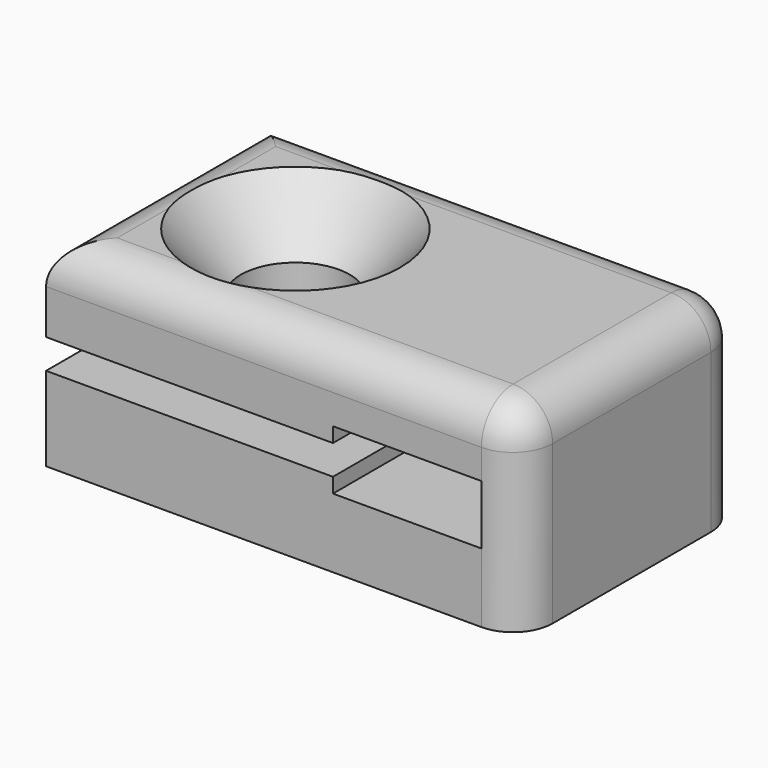
from build123d import *

# Parameters (mm, degrees)
F0_W           = 5
F0_H           = 7
F0_W_2         = 7
F1_DEPTH       = 5
F3_D           = 2.75
F3_CSINK_D     = 5.3
F3_CSINK_ANGLE = 82
F5_DEPTH       = 7
F6_T1_DEPTH    = 12
F6_T3_DEPTH    = 13.5
F6_T5_DEPTH    = 5
F6_T7_DEPTH    = 6.5
F6_S11_W       = 1
F6_S11_H       = 1
F6_T12_DEPTH   = 1
F6_S17_W       = 1
F6_S17_H       = 1
F6_T18_DEPTH   = 1


# Not quite as in the source:
# - a fillet or chamfer that OpenCascade refuses, or shapes differently, is made with other operations: its cross-section is extruded or revolved along the edge and cut away or added


with BuildPart() as f1:
    # F0 (on Top) → F1 (new body)
    with BuildSketch(Plane.XY):
        with Locations((3.5, 0)):
            Rectangle(F0_W, F0_H)
        with Locations((-2.5, 0)):
            Rectangle(F0_W_2, F0_H)
    extrude(amount=-F1_DEPTH)

    # F3 (through all)
    with Locations(Plane.XY):
        with Locations((-2.5, 0)):
            CounterSinkHole(F3_D / 2, F3_CSINK_D / 2, counter_sink_angle=F3_CSINK_ANGLE)

    # F4 (on face) → F5 (cut, through all)
    with BuildSketch(Plane.XZ.offset(3.5)):
        Polygon((1.25, -3.25), (4.9999998882, -3.25), (4.9999998882, -1.75), (1.25, -1.75), (1.25, -2.125), (-6, -2.125), (-6, -2.875), (1.25, -2.875), align=None)
    extrude(amount=-F5_DEPTH, mode=Mode.SUBTRACT)

    # F6: fillet of radius 1 on 6 edges, made by hand

    # F6_s2 → F6_t1 (cut)
    with BuildSketch(Plane.XZ.offset(-6)):
        with BuildLine():
            ThreePointArc((-5, 0), (-5.7071067812, -0.2928932188), (-6, -1))
            Line((-6, -1), (-6, 0))
            Line((-6, 0), (-5, 0))
        make_face()
    extrude(amount=F6_T1_DEPTH, mode=Mode.SUBTRACT)

    # F6_s4 → F6_t3 (cut)
    with BuildSketch(Plane.YZ.offset(-8.5)):
        with BuildLine():
            ThreePointArc((3.5, -1), (3.2071067812, -0.2928932188), (2.5, 0))
            Line((2.5, 0), (3.5, 0))
            Line((3.5, 0), (3.5, -1))
        make_face()
        with BuildLine():
            ThreePointArc((-3.5, -1), (-3.2071067812, -0.2928932188), (-2.5, 0))
            Line((-2.5, 0), (-3.5, 0))
            Line((-3.5, 0), (-3.5, -1))
        make_face()
    extrude(amount=F6_T3_DEPTH, mode=Mode.SUBTRACT)

    # F6_s6 → F6_t5 (cut)
    with BuildSketch(Plane.XZ.offset(-2.5)):
        with BuildLine():
            ThreePointArc((6, -1), (5.7071067812, -0.2928932188), (5, 0))
            Line((5, 0), (6, 0))
            Line((6, 0), (6, -1))
        make_face()
    extrude(amount=F6_T5_DEPTH, mode=Mode.SUBTRACT)

    # F6_s8 → F6_t7 (cut)
    with BuildSketch(Plane.XY.offset(-7.5)):
        with BuildLine():
            ThreePointArc((6, -2.5), (5.7071067812, -3.2071067812), (5, -3.5))
            Line((5, -3.5), (6, -3.5))
            Line((6, -3.5), (6, -2.5))
        make_face()
        with BuildLine():
            ThreePointArc((6, 2.5), (5.7071067812, 3.2071067812), (5, 3.5))
            Line((5, 3.5), (6, 3.5))
            Line((6, 3.5), (6, 2.5))
        make_face()
    extrude(amount=F6_T7_DEPTH, mode=Mode.SUBTRACT)


with BuildPart() as f6_tool10:
    # F6_s11 → F6_t12 (new body)
    with BuildSketch(Plane.YZ.offset(5)):
        with Locations((3, -0.5)):
            Rectangle(F6_S11_W, F6_S11_H)
    extrude(amount=F6_T12_DEPTH)

    # F6_s13 → F6_t14 (revolve, cut)
    with BuildSketch(Plane(origin=(5, 2.5, -1), x_dir=(0, -0.7071067812, -0.7071067812), z_dir=(0, -0.7071067812, 0.7071067812))):
        with BuildLine():
            ThreePointArc((0, -1), (1, 0), (0, 1))
            Line((0, 1), (0, -1))
        make_face()
    revolve(axis=Axis((5, 2.5, -1), (1, 0, 0)), mode=Mode.SUBTRACT)


with BuildPart() as f1_1:
    add(f1.part)

    # F6_t9: cut F6_tool10
    add(f6_tool10.part, mode=Mode.SUBTRACT)


with BuildPart() as f6_tool16:
    # F6_s17 → F6_t18 (new body)
    with BuildSketch(Plane.YZ.offset(5)):
        with Locations((-3, -0.5)):
            Rectangle(F6_S17_W, F6_S17_H)
    extrude(amount=F6_T18_DEPTH)

    # F6_s19 → F6_t20 (revolve, cut)
    with BuildSketch(Plane(origin=(5, -2.5, -1), x_dir=(0, 0.7071067812, -0.7071067812), z_dir=(0, -0.7071067812, -0.7071067812))):
        with BuildLine():
            ThreePointArc((0, -1), (1, 0), (0, 1))
            Line((0, 1), (0, -1))
        make_face()
    revolve(axis=Axis((5, -2.5, -1), (1, 0, 0)), mode=Mode.SUBTRACT)


with BuildPart() as f1_2:
    add(f1_1.part)

    # F6_t15: cut F6_tool16
    add(f6_tool16.part, mode=Mode.SUBTRACT)


solid = f1_2.part
